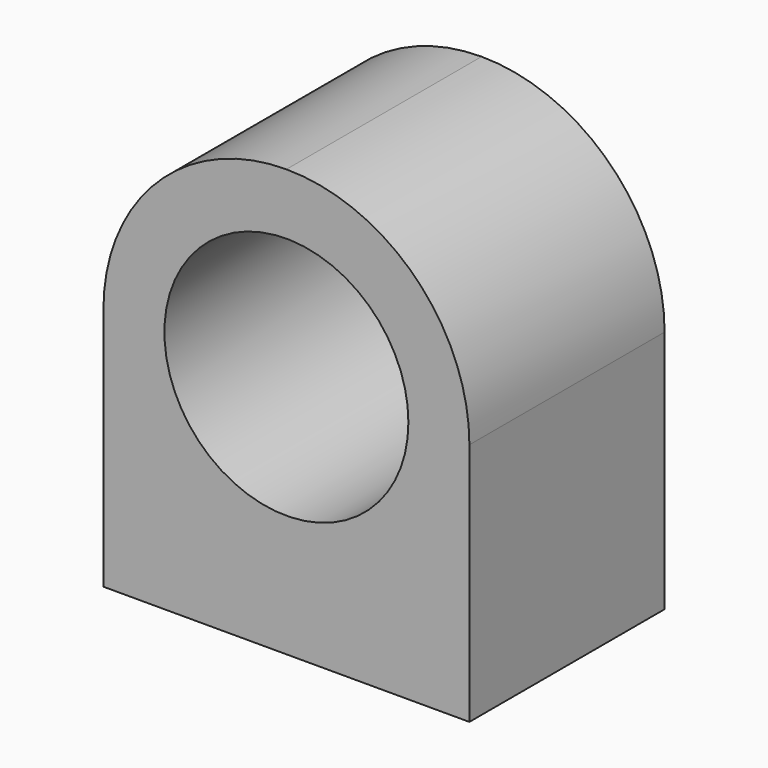
from build123d import *

# Parameters (mm, degrees)
F0_W     = 38.1
F0_H     = 44.45
F1_DEPTH = 25.4
F2_R     = 19.04999
F3_R     = 12.7
F4_DEPTH = 25.401
F5_R     = 3.175
F6_DEPTH = 12.7


# Not quite as in the source:
# - a fillet or chamfer is up to 0.001 mm smaller than in the source, because OpenCascade refuses the exact size


with BuildPart() as f1:
    # F0 (on Front) → F1 (new body)
    with BuildSketch(Plane.XZ):
        with Locations((19.05, 22.225)):
            Rectangle(F0_W, F0_H)
    extrude(amount=F1_DEPTH)

    # F2 (radius 19.05 in the source; OpenCascade refuses exactly that, so slightly less here)
    f2_edges = [f1.edges().sort_by_distance(p)[0] for p in [
        (0, -12.7, 44.45),
        (38.1, -12.7, 44.45),
    ]]
    fillet(f2_edges, radius=F2_R)

    # F3 (on face) → F4 (cut, through all)
    with BuildSketch(Plane.XZ.offset(25.4)):
        with Locations((19.05, 25.4)):
            Circle(F3_R)
    extrude(amount=-F4_DEPTH, mode=Mode.SUBTRACT)

    # F5 (on face) → F6 (cut)
    with BuildSketch(Plane(origin=(0, 0, 0), x_dir=(1, 0, 0), z_dir=(0, 0, -1))):
        with Locations((6.35, 12.7)):
            Circle(F5_R)
        with Locations((31.75, 12.7)):
            Circle(F5_R)
    extrude(amount=-F6_DEPTH, mode=Mode.SUBTRACT)


solid = f1.part
